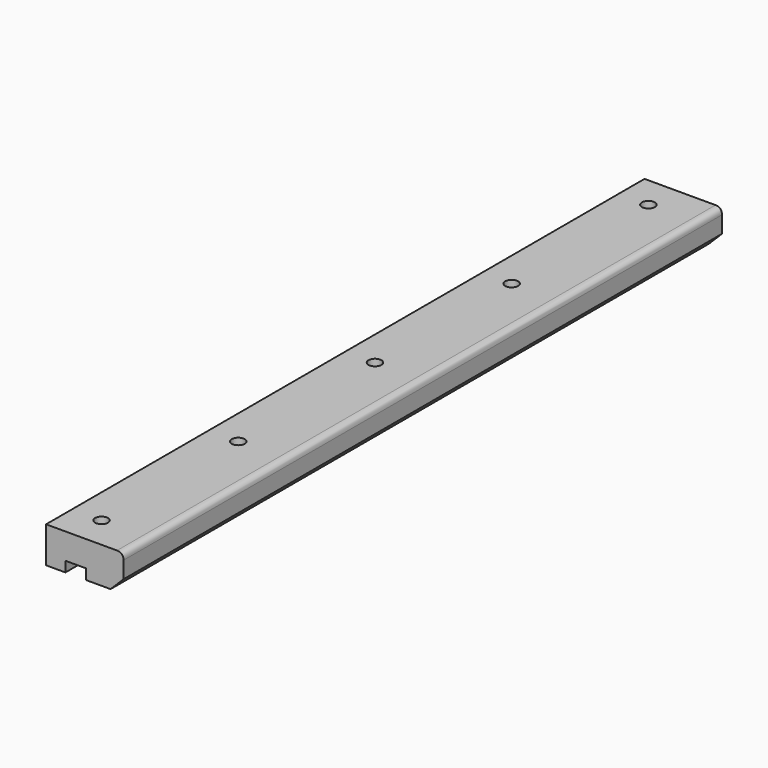
from build123d import *

# Parameters (mm, degrees)
F1_DEPTH    = 580
F2_SIZE2    = 10
F2_SIZE     = 10
F3_T1_DEPTH = 605
F4_R        = 5
F5_DEPTH    = 28.0010001


# Not quite as in the source:
# - a fillet or chamfer that OpenCascade refuses, or shapes differently, is made with other operations: its cross-section is extruded or revolved along the edge and cut away or added


with BuildPart() as f1:
    # F0 (on Front) → F1 (new body)
    with BuildSketch(Plane.XZ):
        Polygon((30, -14), (30, 14), (-30, 14), (-30, -14), (-15, -14), (-15, -6), (1, -6), (1, -14), align=None)
    extrude(amount=F1_DEPTH)

    # F2
    f2_edges = [f1.edges().sort_by_distance(p)[0] for p in [
        (30, -290, -14),
    ]]
    chamfer(f2_edges, length=F2_SIZE, length2=F2_SIZE2)

    # F3: fillet of radius 5 on 1 edges, made by hand

    # F3_s2 → F3_t1 (cut)
    with BuildSketch(Plane.XZ.offset(-12.5)):
        with BuildLine():
            add(Edge.make_bspline(
                [(30, 9), (30, 14), (25, 14)],
                knots=[0, 0, 0, 1, 1, 1], degree=2, weights=[1, 1, 1]))
            Line((25, 14), (30, 14))
            Line((30, 14), (30, 9))
        make_face()
    extrude(amount=F3_T1_DEPTH, mode=Mode.SUBTRACT)

    # F4 (on face) → F5 (cut, through all)
    with BuildSketch(Plane.XY.offset(14)):
        with Locations((-7, -25)):
            Circle(F4_R)
        with Locations((-7, -290)):
            Circle(F4_R)
        with Locations((-7, -157.5)):
            Circle(F4_R)
        with Locations((-7, -422.5)):
            Circle(F4_R)
        with Locations((-7, -555)):
            Circle(F4_R)
    extrude(amount=-F5_DEPTH, mode=Mode.SUBTRACT)


solid = f1.part
